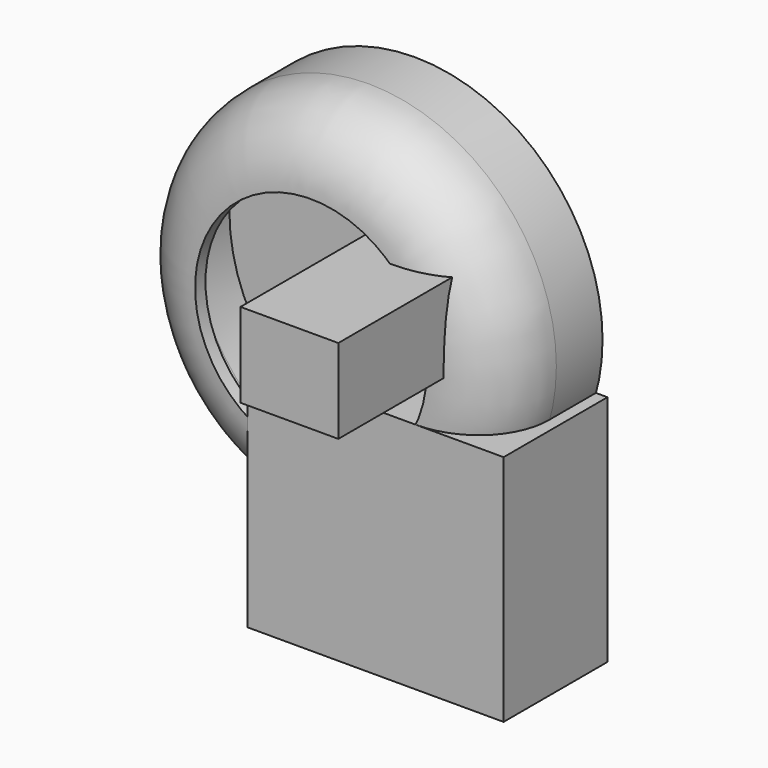
from build123d import *

# Parameters (mm, degrees)
F1_W     = 19.1348660737
F1_H     = 16.5085121989
F2_DEPTH = 25.4
F1_W_2   = 50.0883217901
F1_H_2   = 45.5860048532
F0_R     = 36.7431063658
F3_R     = 14.1038356314
F4_T     = -2.54
F5_DEPTH = 25.4


# Not quite as in the source:
# - a shell that OpenCascade refuses in one call is made with other operations: the cavity is built on its own and cut out


with BuildPart() as f2:
    # F1 (on Front) → F2 (new body)
    with BuildSketch(Plane.XZ):
        with Locations((-27.2015249357, 57.1232028306)):
            Rectangle(F1_W, F1_H)
    extrude(amount=F2_DEPTH)

    # F5 (add): a face of the model
    f5_faces = [f2.faces().sort_by_distance(p)[0] for p in [
        (-27.2015249357, -25.4, 57.1232028306),
    ]]
    extrude(f5_faces, amount=F5_DEPTH)


with BuildPart() as f2b:
    # F1 (on Front) → F2, piece 2 (new body)
    with BuildSketch(Plane.XZ):
        with Locations((-30.6720631197, 16.5085121989)):
            Rectangle(F1_W_2, F1_H_2)
    extrude(amount=F2_DEPTH)


with BuildPart() as f2c:
    # F0 (on Front) → F2, piece 3 (new body)
    with BuildSketch(Plane.XZ):
        with Locations((-43.3348417282, 48.8689467311)):
            Circle(F0_R)
    extrude(amount=F2_DEPTH)

    # F3
    f3_edges = [f2c.edges().sort_by_distance(p)[0] for p in [
        (-80.077948, -25.4, 48.868947),
    ]]
    fillet(f3_edges, radius=F3_R)

    # F4: a shell. OpenCascade refuses it in one call, so the cavity is built on its own and cut out:
    # the body offset inwards by the wall thickness, plus a prism from it out through each open face.
    f4_core = offset(f2c.part, amount=F4_T, mode=Mode.PRIVATE)
    f4_exits = [f4_core.faces().sort_by_distance(p)[0] for p in [
        (-43.334842, -22.86, 48.868947),
    ]]
    add(f4_core, mode=Mode.SUBTRACT)
    extrude(f4_exits, amount=-F4_T, mode=Mode.SUBTRACT)


solid = Compound([f2.part, f2b.part, f2c.part])
